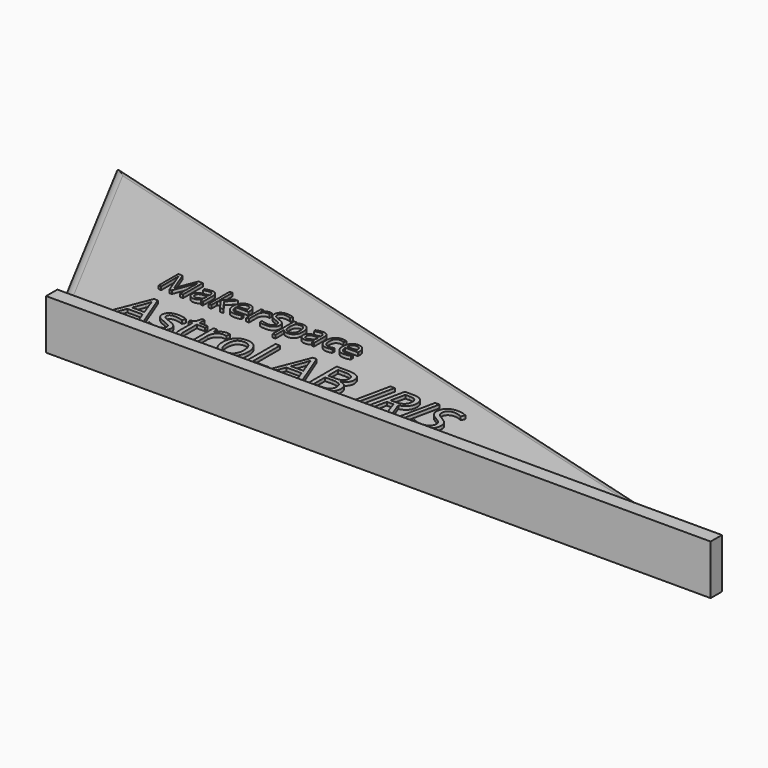
from build123d import *

# Parameters (mm, degrees)
F0_W           = 80
F0_H           = 6
F3_DEPTH       = 1.7
F4_DEPTH       = 1
F5_R           = 0.99999
F7_TEXT_SIZE   = 4.1666666667
F7_TEXT_SIZE_2 = 6.3888888889
F8_DEPTH       = 0.4
F6_TEXT_SIZE   = 4.1666666667
F6_TEXT_SIZE_2 = 6.3888888889
F9_DEPTH       = 0.4


# Not quite as in the source:
# - a fillet or chamfer is up to 0.001 mm smaller than in the source, because OpenCascade refuses the exact size
# - Text() gives the source's letters only with a copy of the font that has no kerning and outlines rounded to 1/6400 em; it was checked with that copy


with BuildPart() as f3:
    # F0 (on Front) → F3 (new body)
    with BuildSketch(Plane.XZ):
        Rectangle(F0_W, F0_H)
    extrude(amount=F3_DEPTH)

    # F2 (on Top) → F4 (join, symmetric)
    with BuildSketch(Plane.XY):
        Polygon((-40, 0), (40, 0), (-54.04621, 26.50857), align=None)
    extrude(amount=F4_DEPTH, both=True)

    # F5 (radius 1 in the source; OpenCascade refuses exactly that, so slightly less here)
    f5_edges = [f3.edges().sort_by_distance(p)[0] for p in [
        (-7.023105, 13.254285, 1),
        (-7.023105, 13.254285, -1),
        (-47.023105, 13.254285, 1),
        (-47.023105, 13.254285, -1),
    ]]
    fillet(f5_edges, radius=F5_R)

    # F7 (on face) → F8 (join)
    with BuildSketch(Plane(origin=(0, 0, -1), x_dir=(1, 0, 0), z_dir=(0, 0, -1))):
        with Locations(Location((-11.5921014331, -9), (0, 0, 180))):
            Text('MakerSpace', F7_TEXT_SIZE, font='Open Sans', text_align=(TextAlign.LEFT, TextAlign.BOTTOM))
        with Locations(Location((-24.5878913636, -2), (0, 0, -180))):
            Text('IRIS', F7_TEXT_SIZE_2, font='Open Sans', font_style=FontStyle.ITALIC, text_align=(TextAlign.LEFT, TextAlign.BOTTOM))
        with Locations(Location((4.4466138447, -2), (0, 0, -180))):
            Text('AstroLAB', F7_TEXT_SIZE_2, font='Open Sans', text_align=(TextAlign.LEFT, TextAlign.BOTTOM))
    extrude(amount=F8_DEPTH)

    # F6 (on face) → F9 (join)
    with BuildSketch(Plane.XY.offset(1)):
        with Locations((-35.4280389331, 9)):
            Text('MakerSpace', F6_TEXT_SIZE, font='Open Sans', text_align=(TextAlign.LEFT, TextAlign.BOTTOM))
        with Locations((-35.4280389331, 2)):
            Text('AstroLAB', F6_TEXT_SIZE_2, font='Open Sans', text_align=(TextAlign.LEFT, TextAlign.BOTTOM))
        with Locations((-6.3935337247, 2)):
            Text('IRIS', F6_TEXT_SIZE_2, font='Open Sans', font_style=FontStyle.ITALIC, text_align=(TextAlign.LEFT, TextAlign.BOTTOM))
    extrude(amount=F9_DEPTH)


solid = f3.part
